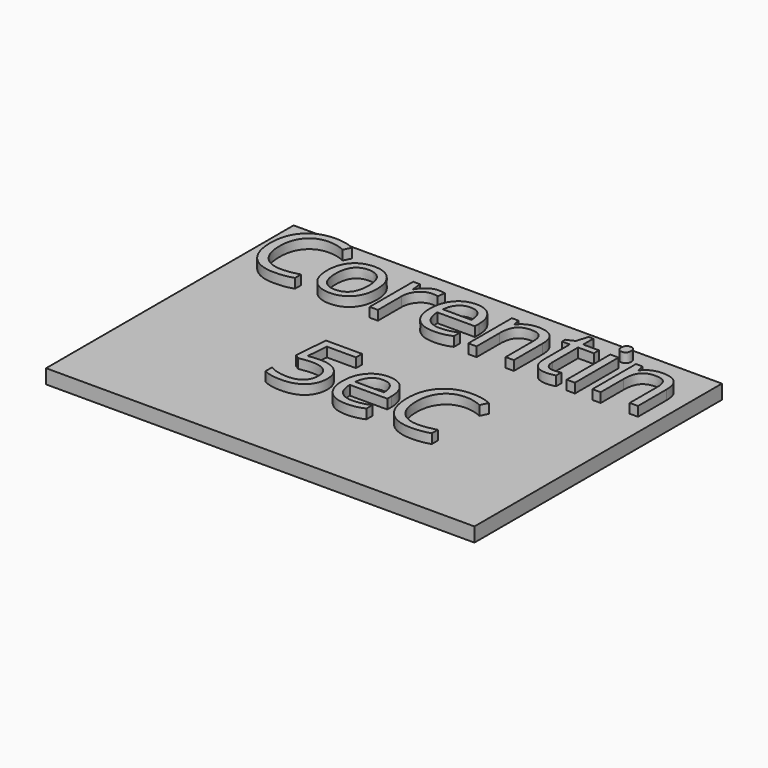
from build123d import *

# Parameters (mm, degrees)
F0_W         = 90
F0_H         = 65
F1_DEPTH     = 3
F2_TEXT_SIZE = 21.3814000466
F3_DEPTH     = 2


# Not quite as in the source:
# - Text() gives the source's letters only with a copy of the font that has no kerning and outlines rounded to 1/6400 em; it was checked with that copy


with BuildPart() as f1:
    # F0 (on Top) → F1 (new body)
    with BuildSketch(Plane.XY):
        with Locations((45, -32.5)):
            Rectangle(F0_W, F0_H)
    extrude(amount=F1_DEPTH)

    # F2 (on face) → F3 (join)
    with BuildSketch(Plane.XY.offset(3)):
        with Locations((2, -17.8176784212)):
            Text('Corentin', F2_TEXT_SIZE, font='Open Sans', text_align=(TextAlign.LEFT, TextAlign.BOTTOM))
        with Locations((29.7791158418, -46.8963824846)):
            Text('5eC', F2_TEXT_SIZE, font='Open Sans', text_align=(TextAlign.LEFT, TextAlign.BOTTOM))
    extrude(amount=F3_DEPTH)


solid = f1.part
